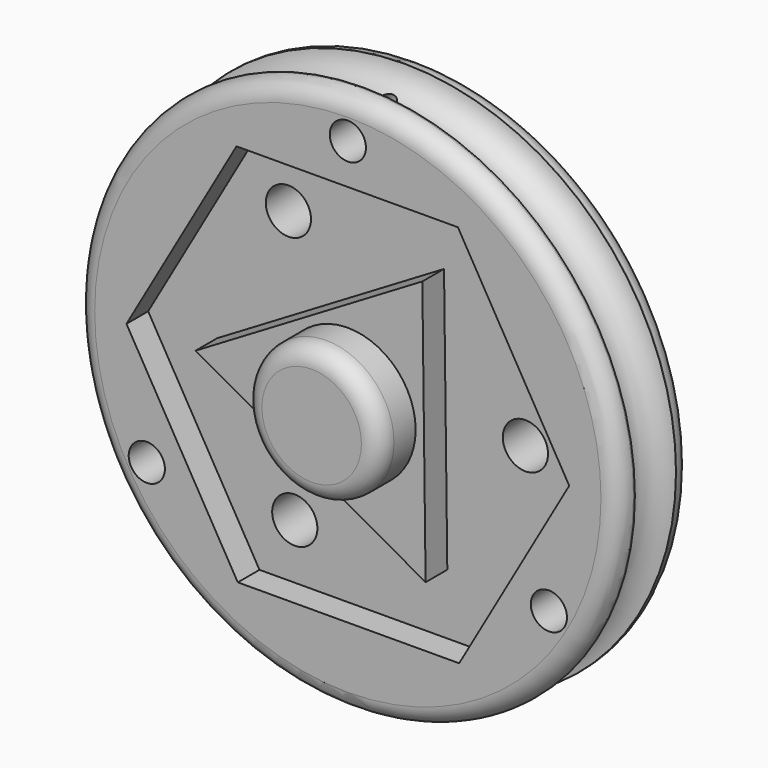
from build123d import *

# Parameters (mm, degrees)
F0_R      = 76.2
F1_DEPTH  = 25.4
F5_D      = 11.43
F6_R      = 19.05
F7_DEPTH  = 12.7
F8_R      = 5.08
F9_R      = 7.2544282258
F11_R     = 5.08
F13_DEPTH = 7.62
F15_DEPTH = 7.62
F16_R     = 6.35
F17_DEPTH = 25.4
F18_R     = 5.08
F19_DEPTH = 25.4


with BuildPart() as f1:
    # F0 (on Front) → F1 (new body)
    with BuildSketch(Plane.XZ):
        Circle(F0_R)
    extrude(amount=F1_DEPTH)

    # F5 (through all)
    with Locations(Plane.XZ.offset(25.4)):
        with Locations((0, 0)):
            Hole(F5_D / 2)

    # F8
    f8_edges = [f1.edges().sort_by_distance(p)[0] for p in [
        (76.2, -12.7, 0),
        (-76.2, 0, 0),
        (-76.2, -25.4, 0),
    ]]
    fillet(f8_edges, radius=F8_R)

    # F9 (on Right) → F10 (revolve, cut)
    with BuildSketch(Plane.YZ):
        with Locations((-12.624304023, 76.8911556739)):
            Circle(F9_R)
    revolve(axis=Axis((0, -25.4, 0), (0, -1, 0)), mode=Mode.SUBTRACT)

    # F12 (on face) → F13 (cut)
    with BuildSketch(Plane.XZ.offset(25.4)):
        Polygon((-30.9163505312, -53.9696626636), (31.2809236348, -53.7591762841), (62.1972741659, 0.2104863795), (30.9163505312, 53.9696626636), (-31.2809236348, 53.7591762841), (-62.1972741659, -0.2104863795), align=None)
    extrude(amount=-F13_DEPTH, mode=Mode.SUBTRACT)

    # F16 (on face) → F17 (cut)
    with BuildSketch(Plane.XZ.offset(25.4)):
        with Locations((-22.7926336229, 37.4113582075)):
            Circle(F16_R)
        with Locations((-21.0028697863, -38.4446788403)):
            Circle(F16_R)
        with Locations((43.7955034092, 1.0333206328)):
            Circle(F16_R)
    extrude(amount=-F17_DEPTH, mode=Mode.SUBTRACT)

    # F18 (on face) → F19 (cut)
    with BuildSketch(Plane.XZ.offset(25.4)):
        with Locations((0, 65.2206302532)):
            Circle(F18_R)
        with Locations((-56.4827226501, -32.6103151266)):
            Circle(F18_R)
        with Locations((56.4827226501, -32.6103151266)):
            Circle(F18_R)
    extrude(amount=-F19_DEPTH, mode=Mode.SUBTRACT)


with BuildPart() as f7:
    # F6 (on face) → F7 (new body)
    with BuildSketch(Plane.XZ.offset(25.4)):
        Circle(F6_R)
    extrude(amount=F7_DEPTH)

    # F11
    f11_edges = [f7.edges().sort_by_distance(p)[0] for p in [
        (-19.05, -38.1, 0),
    ]]
    fillet(f11_edges, radius=F11_R)

    # F14 (on face) → F15 (join)
    with BuildSketch(Plane.XZ.offset(25.4)):
        Polygon((-42.7794071983, -0.5309142646), (21.8494888395, -36.7825962603), (20.9299183588, 37.3135105249), align=None)
    extrude(amount=-F15_DEPTH)


solid = Compound([f1.part, f7.part])
